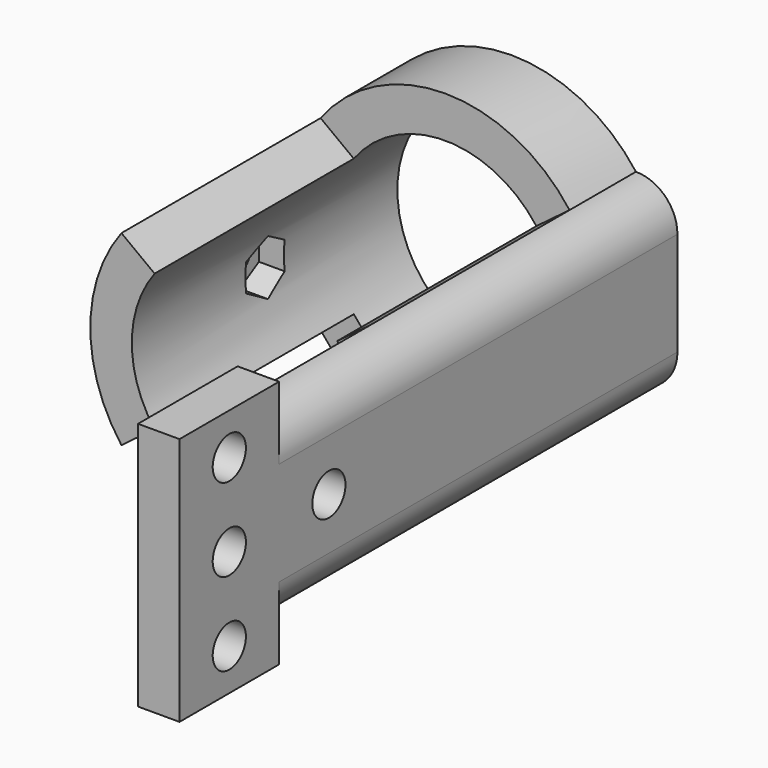
from build123d import *

# Parameters (mm, degrees)
F0_R     = 18.75
F0_R_2   = 13.75
F1_DEPTH = 40
F3_DEPTH = 30
F4_R     = 1.6
F5_DEPTH = 19.750000113
F6_DEPTH = 16.75
F8_R     = 2.5
F9_DEPTH = 5
F10_R    = 4.99999


# Not quite as in the source:
# - a fillet or chamfer is up to 0.001 mm smaller than in the source, because OpenCascade refuses the exact size


with BuildPart() as f1:
    # F0 (on Front) → F1 (new body)
    with BuildSketch(Plane.XZ):
        Circle(F0_R)
        Circle(F0_R_2, mode=Mode.SUBTRACT)
    extrude(amount=F1_DEPTH)

    # F2 (on face) → F3 (cut)
    with BuildSketch(Plane.XZ.offset(40)):
        with BuildLine():
            ThreePointArc((-11, 8.25), (0, 13.75), (11, 8.25))
            Line((11, 8.25), (15, 11.25))
            ThreePointArc((15, 11.25), (0, 18.75), (-15, 11.25))
            Line((-15, 11.25), (-11, 8.25))
        make_face()
        with BuildLine():
            Line((15, -11.25), (11, -8.25))
            ThreePointArc((11, -8.25), (0, -13.75), (-11, -8.25))
            Line((-11, -8.25), (-15, -11.25))
            ThreePointArc((-15, -11.25), (0, -18.75), (15, -11.25))
        make_face()
    extrude(amount=-F3_DEPTH, mode=Mode.SUBTRACT)

    # F4 (on Right) → F5 (cut, up to face)
    with BuildSketch(Plane.YZ):
        with Locations((-20, 0)):
            Circle(F4_R)
    extrude(amount=-F5_DEPTH, mode=Mode.SUBTRACT)

    # F4 (on Right) → F6 (cut)
    with BuildSketch(Plane.YZ):
        Polygon((-22.9, 1.6743157806), (-22.9, -1.6743157806), (-20, -3.3486315613), (-17.1, -1.6743157806), (-17.1, 1.6743157806), (-20, 3.3486315613), align=None)
        with Locations((-20, 0)):
            Circle(F4_R, mode=Mode.SUBTRACT)
    extrude(amount=-F6_DEPTH, mode=Mode.SUBTRACT)

    # F8 (on offset) → F9 (join)
    with BuildSketch(Plane.YZ.offset(20)):
        Polygon((0, 11.25), (-60, 11.25), (-60, 15), (-75, 15), (-75, -15), (-60, -15), (-60, -11.25), (0, -11.25), align=None)
        with Locations((-67.5, -10)):
            Circle(F8_R, mode=Mode.SUBTRACT)
        with Locations((-67.5, 0)):
            Circle(F8_R, mode=Mode.SUBTRACT)
        with Locations((-52.5, 0)):
            Circle(F8_R, mode=Mode.SUBTRACT)
        with Locations((-67.5, 10)):
            Circle(F8_R, mode=Mode.SUBTRACT)
    extrude(amount=-F9_DEPTH)

    # F10 (radius 5 in the source; OpenCascade refuses exactly that, so slightly less here)
    f10_edges = [f1.edges().sort_by_distance(p)[0] for p in [
        (20, -30, 11.25),
        (20, -30, -11.25),
    ]]
    fillet(f10_edges, radius=F10_R)


solid = f1.part
